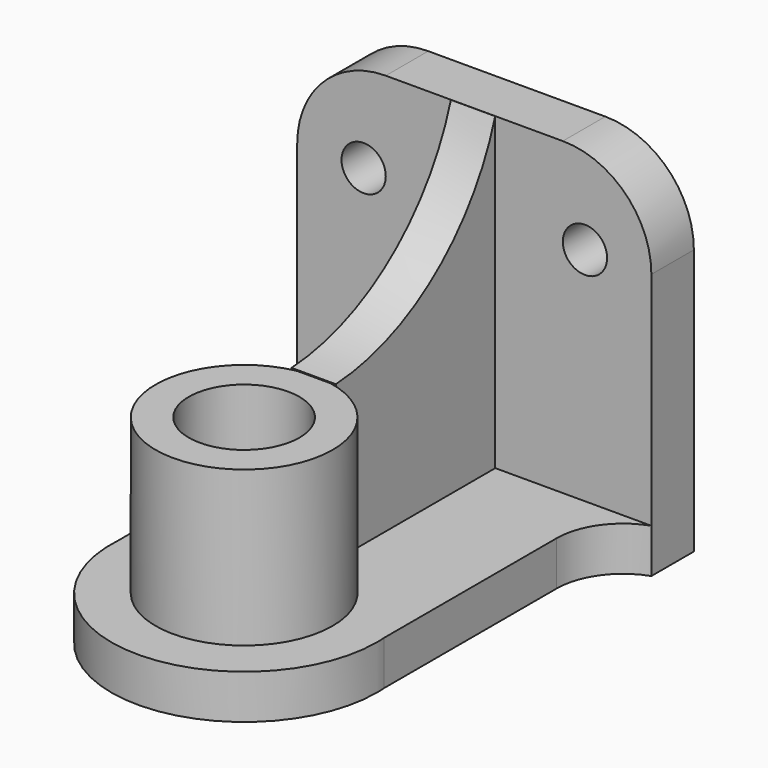
from build123d import *

# Parameters (mm, degrees)
F0_W        = 80
F0_H        = 80
F0_R        = 5
F1_DEPTH    = 12
F2_R        = 20
F3_W        = 80
F3_H        = 10
F4_DEPTH    = 95
F6_DEPTH    = 25
F7_T1_DEPTH = 10
F8_R        = 20
F8_R_2      = 12.5
F9_DEPTH    = 35
F11_DEPTH   = 5


# Not quite as in the source:
# - a fillet or chamfer that OpenCascade refuses, or shapes differently, is made with other operations: its cross-section is extruded or revolved along the edge and cut away or added


with BuildPart() as f1:
    # F0 (on Front) → F1 (new body)
    with BuildSketch(Plane.XZ):
        Rectangle(F0_W, F0_H)
        with Locations((-25, 20)):
            Circle(F0_R, mode=Mode.SUBTRACT)
        with Locations((25, 20)):
            Circle(F0_R, mode=Mode.SUBTRACT)
    extrude(amount=F1_DEPTH)

    # F2
    f2_edges = [f1.edges().sort_by_distance(p)[0] for p in [
        (40, -6, 40),
        (-40, -6, 40),
    ]]
    fillet(f2_edges, radius=F2_R)

    # F3 (on face) → F4 (join)
    with BuildSketch(Plane.XZ.offset(12)):
        with Locations((0, -35)):
            Rectangle(F3_W, F3_H)
    extrude(amount=F4_DEPTH)

    # F5 (on face) → F6 (cut)
    with BuildSketch(Plane.XY.offset(-30)):
        with BuildLine():
            Line((-40, -107), (0, -107))
            ThreePointArc((0, -107), (-21.9575829196, -97.4417355508), (-29.9234068918, -74.857636822))
            Line((-29.9234068918, -74.857636822), (-29.9234068918, -12))
            Line((-29.9234068918, -12), (-40, -12))
            Line((-40, -12), (-40, -107))
        make_face()
        with BuildLine():
            ThreePointArc((29.9234068918, -74.857636822), (29.9808456081, -75.9281340463), (30, -77))
            ThreePointArc((30, -77), (21.2132034356, -98.2132034356), (0, -107))
            Line((0, -107), (40, -107))
            Line((40, -107), (40, -12))
            Line((40, -12), (29.9234068918, -12))
            Line((29.9234068918, -12), (29.9234068918, -74.857636822))
        make_face()
    extrude(amount=-F6_DEPTH, mode=Mode.SUBTRACT)

    # F7: fillet of radius 15 on 2 edges, made by hand

    # F7_s2 → F7_t1 (join)
    with BuildSketch(Plane.XY.offset(-40)):
        with BuildLine():
            ThreePointArc((-40, -12), (-32.6994324281, -17.4756259202), (-29.9234068918, -26.1689824821))
            Line((-29.9234068918, -26.1689824821), (-29.9234068918, -12))
            Line((-29.9234068918, -12), (-40, -12))
        make_face()
        with BuildLine():
            ThreePointArc((40, -12), (32.6994324281, -17.4756259202), (29.9234068918, -26.1689824821))
            Line((29.9234068918, -26.1689824821), (29.9234068918, -12))
            Line((29.9234068918, -12), (40, -12))
        make_face()
    extrude(amount=F7_T1_DEPTH)

    # F8 (on face) → F9 (join)
    with BuildSketch(Plane.XY.offset(-30)):
        with Locations((0, -77)):
            Circle(F8_R)
        with Locations((0, -77)):
            Circle(F8_R_2, mode=Mode.SUBTRACT)
    extrude(amount=F9_DEPTH)

    # F10 (on Right) → F11 (join, symmetric)
    with BuildSketch(Plane.YZ):
        with BuildLine():
            Line((-57.3581678378, -29.785791263), (-12.3581678378, -29.785791263))
            Line((-12.3581678378, -29.785791263), (-12.3581678378, 40.214208737))
            ThreePointArc((-12.3581678378, 40.214208737), (-29.3813213863, 15.6725490137), (-57.3581678378, 5.214208737))
            Line((-57.3581678378, 5.214208737), (-57.3581678378, -29.785791263))
        make_face()
    extrude(amount=F11_DEPTH, both=True)


solid = f1.part
